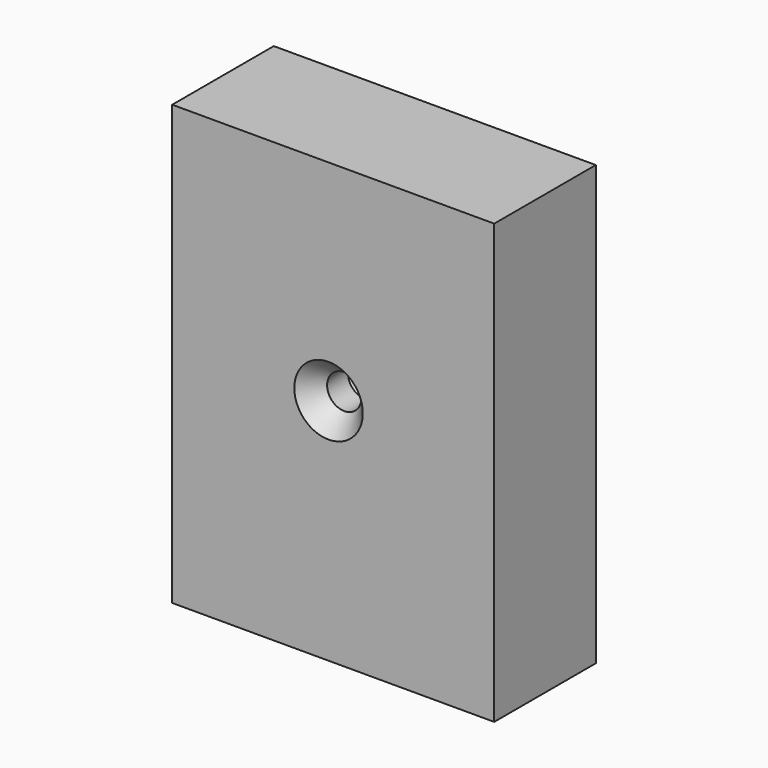
from build123d import *

# Parameters (mm, degrees)
F0_W           = 63.4195655584
F0_H           = 86.4002257586
F1_DEPTH       = 25
F3_D           = 6.7564
F3_DEPTH       = 9
F3_CSINK_D     = 13.4874
F3_CSINK_ANGLE = 82
F3_TIP         = 2.0298273432


# Not quite as in the source:
# - the program builds the solid bodies; features that only make, move or delete a surface that nothing else refers to are left out


with BuildPart() as f1:
    # F0 (on Front) → F1 (new body)
    with BuildSketch(Plane.XZ):
        with Locations((-85.1157233119, 31.1716590077)):
            Rectangle(F0_W, F0_H)
    extrude(amount=F1_DEPTH)

    # F3
    with Locations(Plane.XZ.offset(25)):
        with Locations((-86.0361680388, 33.0585464835)):
            CounterSinkHole(F3_D / 2, F3_CSINK_D / 2, depth=F3_DEPTH, counter_sink_angle=F3_CSINK_ANGLE)
            with Locations((0, 0, -(F3_DEPTH + F3_TIP / 2))):  # 118° drill point
                Cone(0, F3_D / 2, F3_TIP, mode=Mode.SUBTRACT)


solid = f1.part
